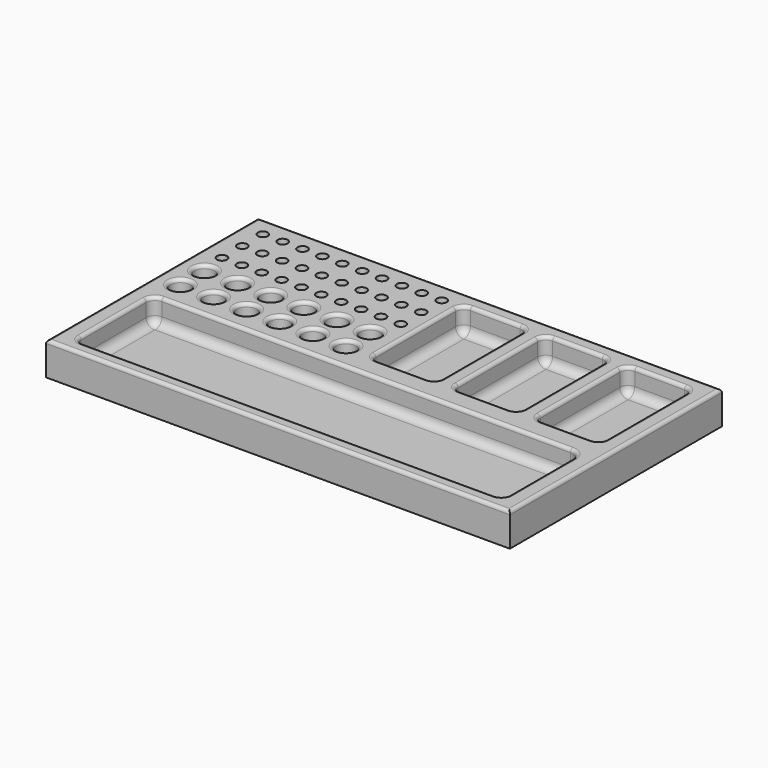
from build123d import *

# Parameters (mm, degrees)
F0_R     = 7.62
F0_R_2   = 3.81
F1_DEPTH = 25.4
F2_DEPTH = 19.05
F3_DEPTH = 12.7
F4_R     = 6.35
F5_R     = 2.54
F6_DEPTH = 21.5


# Not quite as in the source:
# - a feature names something its author has since deleted; it is built from what else it names


with BuildPart() as f1:
    # F0 (on Top) → F1 (new body)
    with BuildSketch(Plane.XY):
        Polygon((295.7100240648, 152.9939571738), (-59.8899759352, 152.9939571738), (-59.8899759352, -50.2060428262), (295.7100240648, -50.2060428262), (295.7100240648, -6.0666222125), (295.7100240648, 49.3900589645), align=None)
        with BuildLine():
            ThreePointArc((282.0640231948, -33.4794739425), (280.2041512554, -37.9696020031), (275.7140231948, -39.8294739425))
            Line((275.7140231948, -39.8294739425), (-39.9671552401, -39.8294739425))
            ThreePointArc((-39.9671552401, -39.8294739425), (-44.4572833006, -37.9696020031), (-46.3171552401, -33.4794739425))
            Line((-46.3171552401, -33.4794739425), (-46.3171552401, 28.7439320236))
            ThreePointArc((-46.3171552401, 28.7439320236), (-44.3613979456, 33.4655478087), (-39.6397821605, 35.4213051032))
            Line((-39.6397821605, 35.4213051032), (273.6397385597, 35.4213051032))
            ThreePointArc((273.6397385597, 35.4213051032), (279.5966073519, 32.9538892602), (282.0640231948, 26.9970204681))
            Line((282.0640231948, 26.9970204681), (282.0640231948, -33.4794739425))
        make_face(mode=Mode.SUBTRACT)
        with Locations((-41.6778475046, 55.7080688701)):
            Circle(F0_R, mode=Mode.SUBTRACT)
        with Locations((-16.2778475046, 55.7080688701)):
            Circle(F0_R, mode=Mode.SUBTRACT)
        with Locations((9.1221524954, 55.7080688701)):
            Circle(F0_R, mode=Mode.SUBTRACT)
        with Locations((-41.6778475046, 78.8220688701)):
            Circle(F0_R, mode=Mode.SUBTRACT)
        with Locations((-16.2778475046, 78.8220688701)):
            Circle(F0_R, mode=Mode.SUBTRACT)
        with Locations((-44.007062912, 98.5187690821)):
            Circle(F0_R_2, mode=Mode.SUBTRACT)
        with Locations((-28.767062912, 98.5187690821)):
            Circle(F0_R_2, mode=Mode.SUBTRACT)
        with Locations((9.1221524954, 78.8220688701)):
            Circle(F0_R, mode=Mode.SUBTRACT)
        with Locations((-13.527062912, 98.5187690821)):
            Circle(F0_R_2, mode=Mode.SUBTRACT)
        with Locations((1.712937088, 98.5187690821)):
            Circle(F0_R_2, mode=Mode.SUBTRACT)
        with Locations((16.952937088, 98.5187690821)):
            Circle(F0_R_2, mode=Mode.SUBTRACT)
        with Locations((34.5221524954, 55.7080688701)):
            Circle(F0_R, mode=Mode.SUBTRACT)
        with Locations((59.9221524954, 55.7080688701)):
            Circle(F0_R, mode=Mode.SUBTRACT)
        with Locations((85.3221524954, 55.7080688701)):
            Circle(F0_R, mode=Mode.SUBTRACT)
        with Locations((34.5221524954, 78.8220688701)):
            Circle(F0_R, mode=Mode.SUBTRACT)
        with Locations((59.9221524954, 78.8220688701)):
            Circle(F0_R, mode=Mode.SUBTRACT)
        with Locations((32.192937088, 98.5187690821)):
            Circle(F0_R_2, mode=Mode.SUBTRACT)
        with Locations((47.432937088, 98.5187690821)):
            Circle(F0_R_2, mode=Mode.SUBTRACT)
        with Locations((62.672937088, 98.5187690821)):
            Circle(F0_R_2, mode=Mode.SUBTRACT)
        with Locations((85.3221524954, 78.8220688701)):
            Circle(F0_R, mode=Mode.SUBTRACT)
        with Locations((77.912937088, 98.5187690821)):
            Circle(F0_R_2, mode=Mode.SUBTRACT)
        with Locations((93.152937088, 98.5187690821)):
            Circle(F0_R_2, mode=Mode.SUBTRACT)
        with Locations((-44.007062912, 118.0767690821)):
            Circle(F0_R_2, mode=Mode.SUBTRACT)
        with Locations((-28.767062912, 118.0767690821)):
            Circle(F0_R_2, mode=Mode.SUBTRACT)
        with Locations((-13.527062912, 118.0767690821)):
            Circle(F0_R_2, mode=Mode.SUBTRACT)
        with Locations((1.712937088, 118.0767690821)):
            Circle(F0_R_2, mode=Mode.SUBTRACT)
        with Locations((16.952937088, 118.0767690821)):
            Circle(F0_R_2, mode=Mode.SUBTRACT)
        with Locations((-44.007062912, 137.6347690821)):
            Circle(F0_R_2, mode=Mode.SUBTRACT)
        with Locations((-28.767062912, 137.6347690821)):
            Circle(F0_R_2, mode=Mode.SUBTRACT)
        with Locations((-13.527062912, 137.6347690821)):
            Circle(F0_R_2, mode=Mode.SUBTRACT)
        with Locations((1.712937088, 137.6347690821)):
            Circle(F0_R_2, mode=Mode.SUBTRACT)
        with Locations((16.952937088, 137.6347690821)):
            Circle(F0_R_2, mode=Mode.SUBTRACT)
        with Locations((32.192937088, 118.0767690821)):
            Circle(F0_R_2, mode=Mode.SUBTRACT)
        with Locations((47.432937088, 118.0767690821)):
            Circle(F0_R_2, mode=Mode.SUBTRACT)
        with Locations((62.672937088, 118.0767690821)):
            Circle(F0_R_2, mode=Mode.SUBTRACT)
        with Locations((77.912937088, 118.0767690821)):
            Circle(F0_R_2, mode=Mode.SUBTRACT)
        with Locations((93.152937088, 118.0767690821)):
            Circle(F0_R_2, mode=Mode.SUBTRACT)
        with Locations((32.192937088, 137.6347690821)):
            Circle(F0_R_2, mode=Mode.SUBTRACT)
        with Locations((47.432937088, 137.6347690821)):
            Circle(F0_R_2, mode=Mode.SUBTRACT)
        with Locations((62.672937088, 137.6347690821)):
            Circle(F0_R_2, mode=Mode.SUBTRACT)
        with Locations((77.912937088, 137.6347690821)):
            Circle(F0_R_2, mode=Mode.SUBTRACT)
        with Locations((93.152937088, 137.6347690821)):
            Circle(F0_R_2, mode=Mode.SUBTRACT)
        with BuildLine():
            Line((112.0100769196, 141.6146457911), (150.1100769196, 141.6146457911))
            ThreePointArc((150.1100769196, 141.6146457911), (154.6002049801, 139.7547738516), (156.4600769196, 135.2646457911))
            Line((156.4600769196, 135.2646457911), (156.4600769196, 59.0646457911))
            ThreePointArc((156.4600769196, 59.0646457911), (154.6002049801, 54.5745177305), (150.1100769196, 52.7146457911))
            Line((150.1100769196, 52.7146457911), (112.0100769196, 52.7146457911))
            ThreePointArc((112.0100769196, 52.7146457911), (107.519948859, 54.5745177305), (105.6600769196, 59.0646457911))
            Line((105.6600769196, 59.0646457911), (105.6600769196, 135.2646457911))
            ThreePointArc((105.6600769196, 135.2646457911), (107.519948859, 139.7547738516), (112.0100769196, 141.6146457911))
        make_face(mode=Mode.SUBTRACT)
        with BuildLine():
            ThreePointArc((213.1020769196, 141.6146457911), (217.5922049801, 139.7547738516), (219.4520769196, 135.2646457911))
            Line((219.4520769196, 135.2646457911), (219.4520769196, 59.0646457911))
            ThreePointArc((219.4520769196, 59.0646457911), (217.5922049801, 54.5745177305), (213.1020769196, 52.7146457911))
            Line((213.1020769196, 52.7146457911), (175.0020769196, 52.7146457911))
            ThreePointArc((175.0020769196, 52.7146457911), (170.511948859, 54.5745177305), (168.6520769196, 59.0646457911))
            Line((168.6520769196, 59.0646457911), (168.6520769196, 135.2646457911))
            ThreePointArc((168.6520769196, 135.2646457911), (170.511948859, 139.7547738516), (175.0020769196, 141.6146457911))
            Line((175.0020769196, 141.6146457911), (213.1020769196, 141.6146457911))
        make_face(mode=Mode.SUBTRACT)
        with BuildLine():
            ThreePointArc((276.0940769196, 141.6146457911), (280.5842049801, 139.7547738516), (282.4440769196, 135.2646457911))
            Line((282.4440769196, 135.2646457911), (282.4440769196, 59.0646457911))
            ThreePointArc((282.4440769196, 59.0646457911), (280.5842049801, 54.5745177305), (276.0940769196, 52.7146457911))
            Line((276.0940769196, 52.7146457911), (237.9940769196, 52.7146457911))
            ThreePointArc((237.9940769196, 52.7146457911), (233.503948859, 54.5745177305), (231.6440769196, 59.0646457911))
            Line((231.6440769196, 59.0646457911), (231.6440769196, 135.2646457911))
            ThreePointArc((231.6440769196, 135.2646457911), (233.503948859, 139.7547738516), (237.9940769196, 141.6146457911))
            Line((237.9940769196, 141.6146457911), (276.0940769196, 141.6146457911))
        make_face(mode=Mode.SUBTRACT)
        with BuildLine():
            Line((-39.9671552401, -39.8294739425), (275.7140231948, -39.8294739425))
            ThreePointArc((275.7140231948, -39.8294739425), (280.2041512554, -37.9696020031), (282.0640231948, -33.4794739425))
            Line((282.0640231948, -33.4794739425), (282.0640231948, 26.9970204681))
            ThreePointArc((282.0640231948, 26.9970204681), (279.5966073519, 32.9538892602), (273.6397385597, 35.4213051032))
            Line((273.6397385597, 35.4213051032), (-39.6397821605, 35.4213051032))
            ThreePointArc((-39.6397821605, 35.4213051032), (-44.3613979456, 33.4655478087), (-46.3171552401, 28.7439320236))
            Line((-46.3171552401, 28.7439320236), (-46.3171552401, -33.4794739425))
            ThreePointArc((-46.3171552401, -33.4794739425), (-44.4572833006, -37.9696020031), (-39.9671552401, -39.8294739425))
        make_face()
        with BuildLine():
            ThreePointArc((156.4600769196, 135.2646457911), (154.6002049801, 139.7547738516), (150.1100769196, 141.6146457911))
            Line((150.1100769196, 141.6146457911), (112.0100769196, 141.6146457911))
            ThreePointArc((112.0100769196, 141.6146457911), (107.519948859, 139.7547738516), (105.6600769196, 135.2646457911))
            Line((105.6600769196, 135.2646457911), (105.6600769196, 59.0646457911))
            ThreePointArc((105.6600769196, 59.0646457911), (107.519948859, 54.5745177305), (112.0100769196, 52.7146457911))
            Line((112.0100769196, 52.7146457911), (150.1100769196, 52.7146457911))
            ThreePointArc((150.1100769196, 52.7146457911), (154.6002049801, 54.5745177305), (156.4600769196, 59.0646457911))
            Line((156.4600769196, 59.0646457911), (156.4600769196, 135.2646457911))
        make_face()
        with BuildLine():
            Line((219.4520769196, 59.0646457911), (219.4520769196, 135.2646457911))
            ThreePointArc((219.4520769196, 135.2646457911), (217.5922049801, 139.7547738516), (213.1020769196, 141.6146457911))
            Line((213.1020769196, 141.6146457911), (175.0020769196, 141.6146457911))
            ThreePointArc((175.0020769196, 141.6146457911), (170.511948859, 139.7547738516), (168.6520769196, 135.2646457911))
            Line((168.6520769196, 135.2646457911), (168.6520769196, 59.0646457911))
            ThreePointArc((168.6520769196, 59.0646457911), (170.511948859, 54.5745177305), (175.0020769196, 52.7146457911))
            Line((175.0020769196, 52.7146457911), (213.1020769196, 52.7146457911))
            ThreePointArc((213.1020769196, 52.7146457911), (217.5922049801, 54.5745177305), (219.4520769196, 59.0646457911))
        make_face()
        with BuildLine():
            Line((282.4440769196, 59.0646457911), (282.4440769196, 135.2646457911))
            ThreePointArc((282.4440769196, 135.2646457911), (280.5842049801, 139.7547738516), (276.0940769196, 141.6146457911))
            Line((276.0940769196, 141.6146457911), (237.9940769196, 141.6146457911))
            ThreePointArc((237.9940769196, 141.6146457911), (233.503948859, 139.7547738516), (231.6440769196, 135.2646457911))
            Line((231.6440769196, 135.2646457911), (231.6440769196, 59.0646457911))
            ThreePointArc((231.6440769196, 59.0646457911), (233.503948859, 54.5745177305), (237.9940769196, 52.7146457911))
            Line((237.9940769196, 52.7146457911), (276.0940769196, 52.7146457911))
            ThreePointArc((276.0940769196, 52.7146457911), (280.5842049801, 54.5745177305), (282.4440769196, 59.0646457911))
        make_face()
        with Locations((34.5221524954, 55.7080688701)):
            Circle(F0_R)
        with Locations((9.1221524954, 55.7080688701)):
            Circle(F0_R)
        with Locations((34.5221524954, 78.8220688701)):
            Circle(F0_R)
        with Locations((9.1221524954, 78.8220688701)):
            Circle(F0_R)
        with Locations((-16.2778475046, 55.7080688701)):
            Circle(F0_R)
        with Locations((-16.2778475046, 78.8220688701)):
            Circle(F0_R)
        with Locations((-41.6778475046, 55.7080688701)):
            Circle(F0_R)
        with Locations((-41.6778475046, 78.8220688701)):
            Circle(F0_R)
        with Locations((85.3221524954, 55.7080688701)):
            Circle(F0_R)
        with Locations((59.9221524954, 55.7080688701)):
            Circle(F0_R)
        with Locations((59.9221524954, 78.8220688701)):
            Circle(F0_R)
        with Locations((85.3221524954, 78.8220688701)):
            Circle(F0_R)
        with Locations((16.952937088, 98.5187690821)):
            Circle(F0_R_2)
        with Locations((62.672937088, 98.5187690821)):
            Circle(F0_R_2)
        with Locations((-13.527062912, 118.0767690821)):
            Circle(F0_R_2)
        with Locations((-13.527062912, 98.5187690821)):
            Circle(F0_R_2)
        with Locations((32.192937088, 98.5187690821)):
            Circle(F0_R_2)
        with Locations((16.952937088, 118.0767690821)):
            Circle(F0_R_2)
        with Locations((47.432937088, 118.0767690821)):
            Circle(F0_R_2)
        with Locations((-44.007062912, 98.5187690821)):
            Circle(F0_R_2)
        with Locations((-44.007062912, 137.6347690821)):
            Circle(F0_R_2)
        with Locations((-44.007062912, 118.0767690821)):
            Circle(F0_R_2)
        with Locations((47.432937088, 137.6347690821)):
            Circle(F0_R_2)
        with Locations((62.672937088, 137.6347690821)):
            Circle(F0_R_2)
        with Locations((32.192937088, 137.6347690821)):
            Circle(F0_R_2)
        with Locations((47.432937088, 98.5187690821)):
            Circle(F0_R_2)
        with Locations((62.672937088, 118.0767690821)):
            Circle(F0_R_2)
        with Locations((1.712937088, 118.0767690821)):
            Circle(F0_R_2)
        with Locations((-13.527062912, 137.6347690821)):
            Circle(F0_R_2)
        with Locations((-28.767062912, 118.0767690821)):
            Circle(F0_R_2)
        with Locations((-28.767062912, 137.6347690821)):
            Circle(F0_R_2)
        with Locations((32.192937088, 118.0767690821)):
            Circle(F0_R_2)
        with Locations((-28.767062912, 98.5187690821)):
            Circle(F0_R_2)
        with Locations((16.952937088, 137.6347690821)):
            Circle(F0_R_2)
        with Locations((1.712937088, 98.5187690821)):
            Circle(F0_R_2)
        with Locations((1.712937088, 137.6347690821)):
            Circle(F0_R_2)
        with Locations((77.912937088, 118.0767690821)):
            Circle(F0_R_2)
        with Locations((93.152937088, 118.0767690821)):
            Circle(F0_R_2)
        with Locations((93.152937088, 137.6347690821)):
            Circle(F0_R_2)
        with Locations((77.912937088, 137.6347690821)):
            Circle(F0_R_2)
        with Locations((77.912937088, 98.5187690821)):
            Circle(F0_R_2)
        with Locations((93.152937088, 98.5187690821)):
            Circle(F0_R_2)
    extrude(amount=-F1_DEPTH)

    # F0 (on Top) → F2 (cut)
    with BuildSketch(Plane.XY):
        with BuildLine():
            ThreePointArc((156.4600769196, 135.2646457911), (154.6002049801, 139.7547738516), (150.1100769196, 141.6146457911))
            Line((150.1100769196, 141.6146457911), (112.0100769196, 141.6146457911))
            ThreePointArc((112.0100769196, 141.6146457911), (107.519948859, 139.7547738516), (105.6600769196, 135.2646457911))
            Line((105.6600769196, 135.2646457911), (105.6600769196, 59.0646457911))
            ThreePointArc((105.6600769196, 59.0646457911), (107.519948859, 54.5745177305), (112.0100769196, 52.7146457911))
            Line((112.0100769196, 52.7146457911), (150.1100769196, 52.7146457911))
            ThreePointArc((150.1100769196, 52.7146457911), (154.6002049801, 54.5745177305), (156.4600769196, 59.0646457911))
            Line((156.4600769196, 59.0646457911), (156.4600769196, 135.2646457911))
        make_face()
        with BuildLine():
            Line((219.4520769196, 59.0646457911), (219.4520769196, 135.2646457911))
            ThreePointArc((219.4520769196, 135.2646457911), (217.5922049801, 139.7547738516), (213.1020769196, 141.6146457911))
            Line((213.1020769196, 141.6146457911), (175.0020769196, 141.6146457911))
            ThreePointArc((175.0020769196, 141.6146457911), (170.511948859, 139.7547738516), (168.6520769196, 135.2646457911))
            Line((168.6520769196, 135.2646457911), (168.6520769196, 59.0646457911))
            ThreePointArc((168.6520769196, 59.0646457911), (170.511948859, 54.5745177305), (175.0020769196, 52.7146457911))
            Line((175.0020769196, 52.7146457911), (213.1020769196, 52.7146457911))
            ThreePointArc((213.1020769196, 52.7146457911), (217.5922049801, 54.5745177305), (219.4520769196, 59.0646457911))
        make_face()
        with BuildLine():
            Line((-39.9671552401, -39.8294739425), (275.7140231948, -39.8294739425))
            ThreePointArc((275.7140231948, -39.8294739425), (280.2041512554, -37.9696020031), (282.0640231948, -33.4794739425))
            Line((282.0640231948, -33.4794739425), (282.0640231948, 26.9970204681))
            ThreePointArc((282.0640231948, 26.9970204681), (279.5966073519, 32.9538892602), (273.6397385597, 35.4213051032))
            Line((273.6397385597, 35.4213051032), (-39.6397821605, 35.4213051032))
            ThreePointArc((-39.6397821605, 35.4213051032), (-44.3613979456, 33.4655478087), (-46.3171552401, 28.7439320236))
            Line((-46.3171552401, 28.7439320236), (-46.3171552401, -33.4794739425))
            ThreePointArc((-46.3171552401, -33.4794739425), (-44.4572833006, -37.9696020031), (-39.9671552401, -39.8294739425))
        make_face()
        with BuildLine():
            Line((282.4440769196, 59.0646457911), (282.4440769196, 135.2646457911))
            ThreePointArc((282.4440769196, 135.2646457911), (280.5842049801, 139.7547738516), (276.0940769196, 141.6146457911))
            Line((276.0940769196, 141.6146457911), (237.9940769196, 141.6146457911))
            ThreePointArc((237.9940769196, 141.6146457911), (233.503948859, 139.7547738516), (231.6440769196, 135.2646457911))
            Line((231.6440769196, 135.2646457911), (231.6440769196, 59.0646457911))
            ThreePointArc((231.6440769196, 59.0646457911), (233.503948859, 54.5745177305), (237.9940769196, 52.7146457911))
            Line((237.9940769196, 52.7146457911), (276.0940769196, 52.7146457911))
            ThreePointArc((276.0940769196, 52.7146457911), (280.5842049801, 54.5745177305), (282.4440769196, 59.0646457911))
        make_face()
    extrude(amount=-F2_DEPTH, mode=Mode.SUBTRACT)

    # F0 (on Top) → F3 (cut)
    with BuildSketch(Plane.XY):
        with Locations((-41.6778475046, 78.8220688701)):
            Circle(F0_R)
        with Locations((-16.2778475046, 78.8220688701)):
            Circle(F0_R)
        with Locations((9.1221524954, 78.8220688701)):
            Circle(F0_R)
        with Locations((34.5221524954, 78.8220688701)):
            Circle(F0_R)
        with Locations((34.5221524954, 55.7080688701)):
            Circle(F0_R)
        with Locations((9.1221524954, 55.7080688701)):
            Circle(F0_R)
        with Locations((-16.2778475046, 55.7080688701)):
            Circle(F0_R)
        with Locations((-41.6778475046, 55.7080688701)):
            Circle(F0_R)
        with Locations((59.9221524954, 78.8220688701)):
            Circle(F0_R)
        with Locations((85.3221524954, 78.8220688701)):
            Circle(F0_R)
        with Locations((59.9221524954, 55.7080688701)):
            Circle(F0_R)
        with Locations((85.3221524954, 55.7080688701)):
            Circle(F0_R)
    extrude(amount=-F3_DEPTH, mode=Mode.SUBTRACT)

    # F4
    f4_edges = [f1.edges().sort_by_distance(p)[0] for p in [
        (154.600205, 139.754774, -19.05),
        (131.060077, 141.614646, -19.05),
        (107.519949, 139.754774, -19.05),
        (105.660077, 97.164646, -19.05),
        (107.519949, 54.574518, -19.05),
        (131.060077, 52.714646, -19.05),
        (154.600205, 54.574518, -19.05),
        (156.460077, 97.164646, -19.05),
        (219.452077, 97.164646, -19.05),
        (217.592205, 139.754774, -19.05),
        (194.052077, 141.614646, -19.05),
        (170.511949, 139.754774, -19.05),
        (168.652077, 97.164646, -19.05),
        (170.511949, 54.574518, -19.05),
        (194.052077, 52.714646, -19.05),
        (217.592205, 54.574518, -19.05),
        (117.873434, -39.829474, -19.05),
        (280.204151, -37.969602, -19.05),
        (282.064023, -3.241227, -19.05),
        (279.596607, 32.953889, -19.05),
        (116.999978, 35.421305, -19.05),
        (-44.361398, 33.465548, -19.05),
        (-46.317155, -2.367771, -19.05),
        (-44.457283, -37.969602, -19.05),
        (257.044077, 141.614646, -19.05),
    ]]
    fillet(f4_edges, radius=F4_R)

    # F5
    f5_edges = [f1.edges().sort_by_distance(p)[0] for p in [
        (117.910024, 152.993957, 0),
        (295.710024, 51.393957, 0),
        (-59.889976, 51.393957, 0),
        (117.910024, -50.206043, 0),
        (117.873434, -39.829474, 0),
        (-44.457283, -37.969602, 0),
        (280.204151, -37.969602, 0),
        (-46.317155, -2.367771, 0),
        (282.064023, -3.241227, 0),
        (-44.361398, 33.465548, 0),
        (279.596607, 32.953889, 0),
        (116.999978, 35.421305, 0),
        (-49.297848, 55.708069, 0),
        (-23.897848, 55.708069, 0),
        (1.502152, 55.708069, 0),
        (-49.297848, 78.822069, 0),
        (-23.897848, 78.822069, 0),
        (1.502152, 78.822069, 0),
        (26.902152, 55.708069, 0),
        (52.302152, 55.708069, 0),
        (77.702152, 55.708069, 0),
        (26.902152, 78.822069, 0),
        (52.302152, 78.822069, 0),
        (77.702152, 78.822069, 0),
        (154.600205, 139.754774, 0),
        (156.460077, 97.164646, 0),
        (131.060077, 141.614646, 0),
        (154.600205, 54.574518, 0),
        (107.519949, 139.754774, 0),
        (131.060077, 52.714646, 0),
        (105.660077, 97.164646, 0),
        (107.519949, 54.574518, 0),
        (219.452077, 97.164646, 0),
        (217.592205, 54.574518, 0),
        (217.592205, 139.754774, 0),
        (194.052077, 52.714646, 0),
        (194.052077, 141.614646, 0),
        (170.511949, 54.574518, 0),
        (170.511949, 139.754774, 0),
        (168.652077, 97.164646, 0),
        (257.044077, 52.714646, 0),
        (233.503949, 54.574518, 0),
        (280.584205, 54.574518, 0),
        (231.644077, 97.164646, 0),
        (282.444077, 97.164646, 0),
        (233.503949, 139.754774, 0),
        (280.584205, 139.754774, 0),
        (257.044077, 141.614646, 0),
    ]]
    fillet(f5_edges, radius=F5_R)

    # F0 (on Top) → F6 (cut)
    with BuildSketch(Plane.XY):
        with Locations((-44.007062912, 137.6347690821)):
            Circle(F0_R_2)
        with Locations((-44.007062912, 118.0767690821)):
            Circle(F0_R_2)
        with Locations((-44.007062912, 98.5187690821)):
            Circle(F0_R_2)
        with Locations((-28.767062912, 98.5187690821)):
            Circle(F0_R_2)
        with Locations((-28.767062912, 118.0767690821)):
            Circle(F0_R_2)
        with Locations((-13.527062912, 118.0767690821)):
            Circle(F0_R_2)
        with Locations((-13.527062912, 98.5187690821)):
            Circle(F0_R_2)
        with Locations((1.712937088, 98.5187690821)):
            Circle(F0_R_2)
        with Locations((1.712937088, 118.0767690821)):
            Circle(F0_R_2)
        with Locations((16.952937088, 118.0767690821)):
            Circle(F0_R_2)
        with Locations((16.952937088, 98.5187690821)):
            Circle(F0_R_2)
        with Locations((32.192937088, 118.0767690821)):
            Circle(F0_R_2)
        with Locations((32.192937088, 98.5187690821)):
            Circle(F0_R_2)
        with Locations((-28.767062912, 137.6347690821)):
            Circle(F0_R_2)
        with Locations((-13.527062912, 137.6347690821)):
            Circle(F0_R_2)
        with Locations((1.712937088, 137.6347690821)):
            Circle(F0_R_2)
        with Locations((16.952937088, 137.6347690821)):
            Circle(F0_R_2)
        with Locations((32.192937088, 137.6347690821)):
            Circle(F0_R_2)
        with Locations((47.432937088, 137.6347690821)):
            Circle(F0_R_2)
        with Locations((62.672937088, 137.6347690821)):
            Circle(F0_R_2)
        with Locations((47.432937088, 118.0767690821)):
            Circle(F0_R_2)
        with Locations((62.672937088, 118.0767690821)):
            Circle(F0_R_2)
        with Locations((47.432937088, 98.5187690821)):
            Circle(F0_R_2)
        with Locations((62.672937088, 98.5187690821)):
            Circle(F0_R_2)
        with Locations((77.912937088, 98.5187690821)):
            Circle(F0_R_2)
        with Locations((77.912937088, 118.0767690821)):
            Circle(F0_R_2)
        with Locations((77.912937088, 137.6347690821)):
            Circle(F0_R_2)
        with Locations((93.152937088, 137.6347690821)):
            Circle(F0_R_2)
        with Locations((93.152937088, 118.0767690821)):
            Circle(F0_R_2)
        with Locations((93.152937088, 98.5187690821)):
            Circle(F0_R_2)
    extrude(amount=-F6_DEPTH, mode=Mode.SUBTRACT)


solid = f1.part
